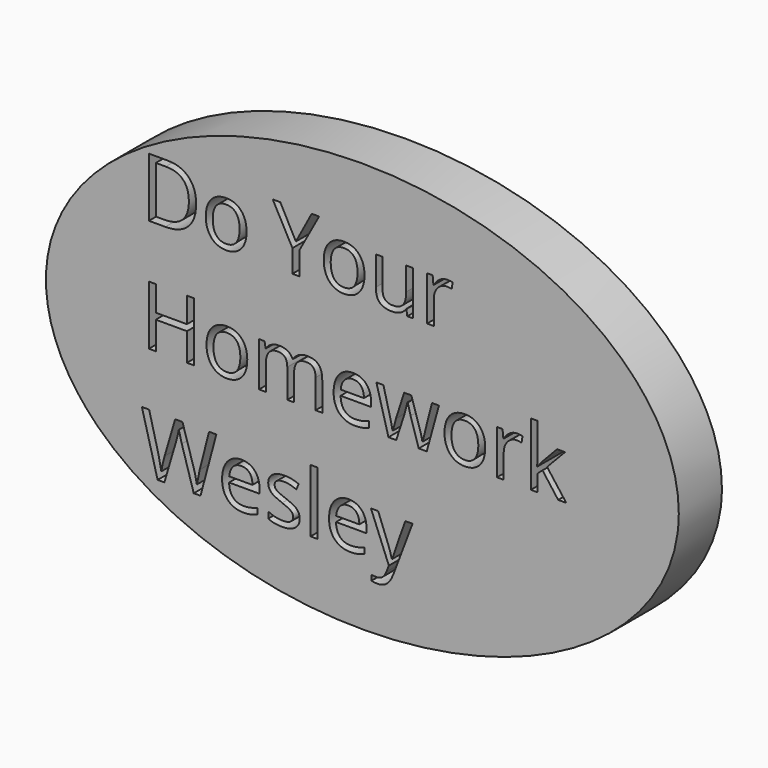
from build123d import *

# Parameters (mm, degrees)
F1_DEPTH     = 12.7
F2_TEXT_SIZE = 19.5131292313
F3_DEPTH     = 25.4


# Not quite as in the source:
# - Text() gives the source's letters only with a copy of the font that has no kerning and outlines rounded to 1/6400 em; it was checked with that copy


with BuildPart() as f1:
    # F0 (on Front) → F1 (new body)
    with BuildSketch(Plane.XZ):
        with BuildLine():
            add(Edge.make_bspline(
                [(75.9940594435, 0), (75.9940594435, 83.6868688685), (-35.8345971908, 41.8434344342), (-147.6632538252, 0), (-35.8345971908, -41.8434344342), (75.9940594435, -83.6868688685), (75.9940594435, 0)],
                knots=[0, 0, 0, 2.0943951024, 2.0943951024, 4.1887902048, 4.1887902048, 6.2831853072, 6.2831853072, 6.2831853072], degree=2, weights=[1, 0.5, 1, 0.5, 1, 0.5, 1]))
        make_face()
    extrude(amount=F1_DEPTH)

    # F2 (on Front) → F3 (cut)
    with BuildSketch(Plane.XZ):
        with Locations((-50.7570029496, 20.0675190922)):
            Text('Do Your', F2_TEXT_SIZE, font='Open Sans', text_align=(TextAlign.LEFT, TextAlign.BOTTOM))
        with Locations((-50.7570029496, -6.4703366623)):
            Text('Homework', F2_TEXT_SIZE, font='Open Sans', text_align=(TextAlign.LEFT, TextAlign.BOTTOM))
        with Locations((-50.7570029496, -33.0081924169)):
            Text('Wesley', F2_TEXT_SIZE, font='Open Sans', text_align=(TextAlign.LEFT, TextAlign.BOTTOM))
    extrude(amount=F3_DEPTH, mode=Mode.SUBTRACT)


solid = f1.part
